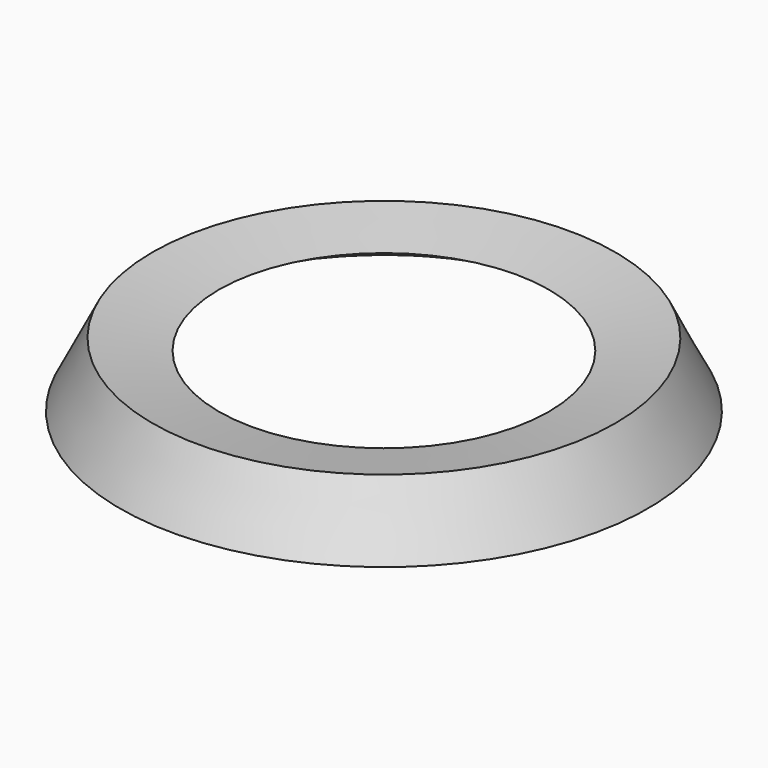
from build123d import *


# Not quite as in the source:
# - a feature of the source that left no trace in its solid (it failed there, or was rolled back) is left out


with BuildPart() as f1:
    # F0 (on Front) → F1 (revolve)
    with BuildSketch(Plane.XZ):
        with BuildLine():
            ThreePointArc((-161.10966, -59.8573098), (-130.7493020114, -43.9701584499), (-100.759768, -27.393646))
            Line((-100.759768, -27.393646), (-141.309598, -20.4573886))
            Line((-141.309598, -20.4573886), (-161.10966, -59.8573098))
        make_face()
    revolve(axis=Axis((0, 0, -50.3860435), (0, 0, -1)))


solid = f1.part
